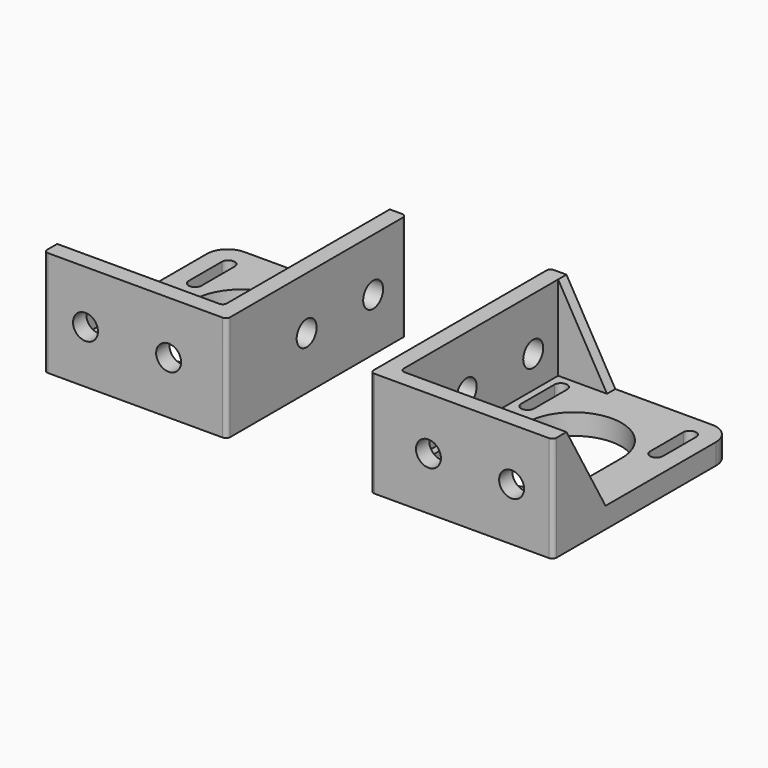
from build123d import *

# Parameters (mm, degrees)
F0_W        = 42.5
F0_H        = 52.5
F0_H_2      = 1.5
F1_DEPTH    = 5
F2_W        = 2.5
F2_H        = 11.75
F2_W_2      = 11.75
F2_H_2      = 2.5
F3_DEPTH    = 20.4
F4_R        = 3
F5_DEPTH    = 4.001
F6_R        = 3
F7_DEPTH    = 4.001
F8_R        = 1
F9_R        = 5
F10_SIZE2   = 11.74999
F10_SIZE    = 20.39999
F10_2_SIZE2 = 11.74999
F10_2_SIZE  = 20.39999


# Not quite as in the source:
# - a fillet or chamfer is up to 0.001 mm smaller than in the source, because OpenCascade refuses the exact size


with BuildPart() as f1:
    # F0 (on Top) → F1 (new body)
    with BuildSketch(Plane.XY):
        with Locations((0, 5)):
            Rectangle(F0_W, F0_H)
        with BuildLine():
            ThreePointArc((-13.95, -15.5), (-15.5, -17.05), (-17.05, -15.5))
            Line((-17.05, -15.5), (-17.05, -5.5))
            ThreePointArc((-17.05, -5.5), (-15.5, -3.95), (-13.95, -5.5))
            Line((-13.95, -5.5), (-13.95, -15.5))
        make_face(mode=Mode.SUBTRACT)
        with BuildLine():
            Line((13.95, -15.5), (13.95, -5.5))
            ThreePointArc((13.95, -5.5), (15.5, -3.95), (17.05, -5.5))
            Line((17.05, -5.5), (17.05, -15.5))
            ThreePointArc((17.05, -15.5), (15.5, -17.05), (13.95, -15.5))
        make_face(mode=Mode.SUBTRACT)
        with BuildLine():
            ThreePointArc((11.5, 0), (0, -11.5), (-11.5, 0))
            Line((-11.5, 0), (-11.5, 10))
            ThreePointArc((-11.5, 10), (0, 21.5), (11.5, 10))
            Line((11.5, 10), (11.5, 0))
        make_face(mode=Mode.SUBTRACT)
        with BuildLine():
            ThreePointArc((-13.95, 15.5), (-15.5, 13.95), (-17.05, 15.5))
            Line((-17.05, 15.5), (-17.05, 25.5))
            ThreePointArc((-17.05, 25.5), (-15.5, 27.05), (-13.95, 25.5))
            Line((-13.95, 25.5), (-13.95, 15.5))
        make_face(mode=Mode.SUBTRACT)
        with BuildLine():
            Line((17.05, 25.5), (17.05, 15.5))
            ThreePointArc((17.05, 15.5), (15.5, 13.95), (13.95, 15.5))
            Line((13.95, 15.5), (13.95, 25.5))
            ThreePointArc((13.95, 25.5), (15.5, 27.05), (17.05, 25.5))
        make_face(mode=Mode.SUBTRACT)
        Polygon((22.75, 31.25), (21.25, 31.25), (21.25, -21.25), (21.25, -22.75), (22.75, -22.75), align=None)
        with Locations((0, -22)):
            Rectangle(F0_W, F0_H_2)
    extrude(amount=F1_DEPTH)

    # F2 (on face) → F3 (join)
    with BuildSketch(Plane.XY.offset(5)):
        Polygon((-21.25, -18.75), (-21.25, -22.75), (22.75, -22.75), (22.75, -18.75), (18.75, -18.75), (-18.75, -18.75), align=None)
        with Locations((-20, -12.875)):
            Rectangle(F2_W, F2_H)
        Polygon((18.75, -18.75), (22.75, -18.75), (22.75, 31.25), (18.75, 31.25), (18.75, 28.75), align=None)
        with Locations((12.875, 30)):
            Rectangle(F2_W_2, F2_H_2)
    extrude(amount=F3_DEPTH)

    # F4 (on face) → F5 (cut, through all)
    with BuildSketch(Plane(origin=(0, -18.75, 0), x_dir=(-1, 0, 0), z_dir=(0, 1, 0))):
        with Locations((11.25, 12.7)):
            Circle(F4_R)
        with Locations((-8.75, 12.7)):
            Circle(F4_R)
    extrude(amount=-F5_DEPTH, mode=Mode.SUBTRACT)

    # F6 (on face) → F7 (cut, through all)
    with BuildSketch(Plane(origin=(18.75, 0, 0), x_dir=(0, -1, 0), z_dir=(-1, 0, 0))):
        with Locations((-1.25, 12.7)):
            Circle(F6_R)
        with Locations((-21.25, 12.7)):
            Circle(F6_R)
    extrude(amount=-F7_DEPTH, mode=Mode.SUBTRACT)

    # F8
    f8_edges = [f1.edges().sort_by_distance(p)[0] for p in [
        (-21.25, -22.75, 12.7),
        (22.75, -22.75, 12.7),
        (22.75, 31.25, 12.7),
        (18.75, -18.75, 15.2),
    ]]
    fillet(f8_edges, radius=F8_R)

    # F9
    f9_edges = [f1.edges().sort_by_distance(p)[0] for p in [
        (-21.25, 31.25, 2.5),
    ]]
    fillet(f9_edges, radius=F9_R)

    # F10 (size 20.4 and 11.75 in the source; OpenCascade refuses exactly that, so slightly less here)
    f10_edges = [f1.edges().sort_by_distance(p)[0] for p in [
        (-20, -7, 25.4),
    ]]
    f10_side = f1.faces().sort_by_distance((-20, -7, 15.2))[0]
    chamfer(f10_edges, length=F10_SIZE, length2=F10_SIZE2, reference=f10_side)

    # F10#2 (size 20.4 and 11.75 in the source; OpenCascade refuses exactly that, so slightly less here)
    f10_2_edges = [f1.edges().sort_by_distance(p)[0] for p in [
        (7, 30, 25.4),
    ]]
    f10_2_side = f1.faces().sort_by_distance((7, 30, 15.2))[0]
    chamfer(f10_2_edges, length=F10_2_SIZE, length2=F10_2_SIZE2, reference=f10_2_side)


with BuildPart() as f11_1:
    # F11: instance of F1
    add(f1.part.mirror(Plane.YZ))


with BuildPart() as f11_1_1:
    # F12: moved
    add(f11_1.part.moved(Location((80, 0, 0))))


solid = Compound([f1.part, f11_1_1.part])
